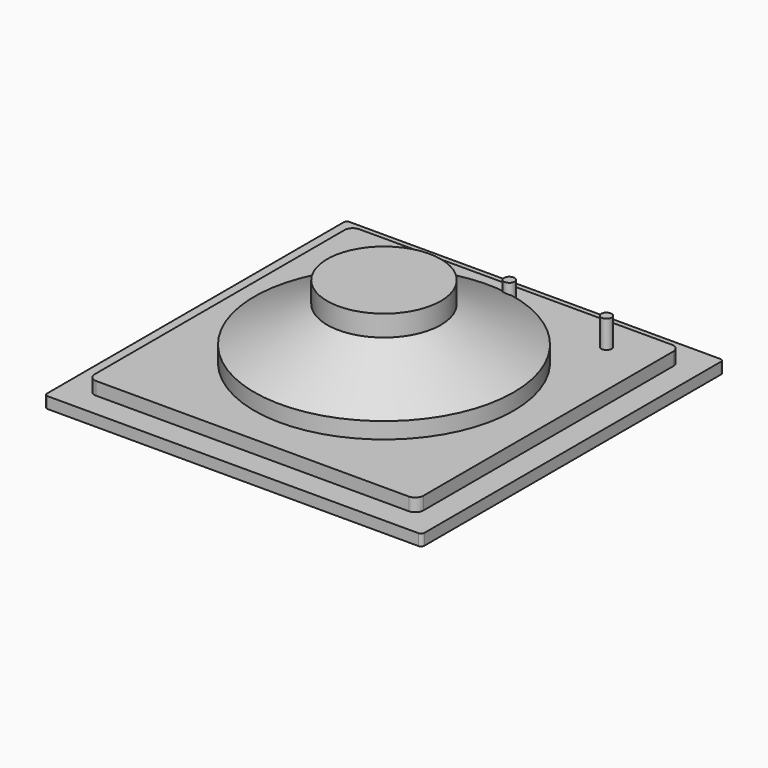
from build123d import *

# Parameters (mm, degrees)
F0_R      = 80.0681985748
F1_DEPTH  = 15
F2_DEPTH  = 7
F7_START  = 25
F0_R_2    = 35.086234683
F7_DEPTH  = 22
F8_DEPTH  = 25
F8_FACE_R = 80.0681985748
F7_FACE_R = 35.086234683
F10_DEPTH = 13
F6_R      = 3.2141015645
F11_DEPTH = 32
F6_R_2    = 3.2204856396


# Not quite as in the source:
# - the program builds the solid bodies; features that only make, move or delete a surface that nothing else refers to are left out


with BuildPart() as f1:
    # F0 (on Top) → F1 (new body)
    with BuildSketch(Plane.XY):
        with BuildLine():
            ThreePointArc((-96.5, 101.5), (-100.0355339059, 100.0355339059), (-101.5, 96.5))
            Line((-101.5, 96.5), (-101.5, -96.5))
            ThreePointArc((-101.5, -96.5), (-100.0355339059, -100.0355339059), (-96.5, -101.5))
            Line((-96.5, -101.5), (96.5, -101.5))
            ThreePointArc((96.5, -101.5), (100.0355339059, -100.0355339059), (101.5, -96.5))
            Line((101.5, -96.5), (101.5, 96.5))
            ThreePointArc((101.5, 96.5), (100.0355339059, 100.0355339059), (96.5, 101.5))
            Line((96.5, 101.5), (-96.5, 101.5))
        make_face()
        Circle(F0_R, mode=Mode.SUBTRACT)
    extrude(amount=F1_DEPTH)

    # F0 (on Top) → F2 (join)
    with BuildSketch(Plane.XY):
        with BuildLine():
            Line((114.5, 116.5), (-114.5, 116.5))
            ThreePointArc((-114.5, 116.5), (-115.9142135624, 115.9142135624), (-116.5, 114.5))
            Line((-116.5, 114.5), (-116.5, -114.5))
            ThreePointArc((-116.5, -114.5), (-115.9142135624, -115.9142135624), (-114.5, -116.5))
            Line((-114.5, -116.5), (114.5, -116.5))
            ThreePointArc((114.5, -116.5), (115.9142135624, -115.9142135624), (116.5, -114.5))
            Line((116.5, -114.5), (116.5, 114.5))
            ThreePointArc((116.5, 114.5), (115.9142135624, 115.9142135624), (114.5, 116.5))
        make_face()
        with BuildLine():
            Line((-101.5, -96.5), (-101.5, 96.5))
            ThreePointArc((-101.5, 96.5), (-100.0355339059, 100.0355339059), (-96.5, 101.5))
            Line((-96.5, 101.5), (96.5, 101.5))
            ThreePointArc((96.5, 101.5), (100.0355339059, 100.0355339059), (101.5, 96.5))
            Line((101.5, 96.5), (101.5, -96.5))
            ThreePointArc((101.5, -96.5), (100.0355339059, -100.0355339059), (96.5, -101.5))
            Line((96.5, -101.5), (-96.5, -101.5))
            ThreePointArc((-96.5, -101.5), (-100.0355339059, -100.0355339059), (-101.5, -96.5))
        make_face(mode=Mode.SUBTRACT)
    extrude(amount=F2_DEPTH)


with BuildPart() as f7:
    # F0 (on Top) → F7 (new body)
    with BuildSketch(Plane.XY.offset(F7_START)):
        Circle(F0_R_2)
    extrude(amount=F7_DEPTH)


with BuildPart() as f8:
    # F0 (on Top) → F8 (new body)
    with BuildSketch(Plane.XY):
        Circle(F0_R)
        Circle(F0_R_2, mode=Mode.SUBTRACT)
        Circle(F0_R_2)
    extrude(amount=F8_DEPTH)


with BuildPart() as f9:
    # F8_face (on face) → F9 section 0
    with BuildSketch(Plane.XY.offset(25)):
        Circle(F8_FACE_R)
    # F7_face (on face) → F9 section 1
    with BuildSketch(Plane.XY.offset(47)):
        Circle(F7_FACE_R)
    loft()


with BuildPart() as f10:
    # F10 (new): a face of the model
    f10_faces = [f7.part.faces().sort_by_distance(p)[0] for p in [
        (0, 0, 47),
    ]]
    extrude(f10_faces, amount=F10_DEPTH)


with BuildPart() as f11:
    # F6 (on Top) → F11 (new body)
    with BuildSketch(Plane.XY):
        with Locations((13.3781218901, 79.9919366837)):
            Circle(F6_R)
    extrude(amount=F11_DEPTH)


with BuildPart() as f11b:
    # F6 (on Top) → F11, piece 2 (new body)
    with BuildSketch(Plane.XY):
        with Locations((73.3781218901, 79.9919366837)):
            Circle(F6_R_2)
    extrude(amount=F11_DEPTH)


solid = Compound([f1.part, f7.part, f8.part, f9.part, f10.part, f11.part, f11b.part])
